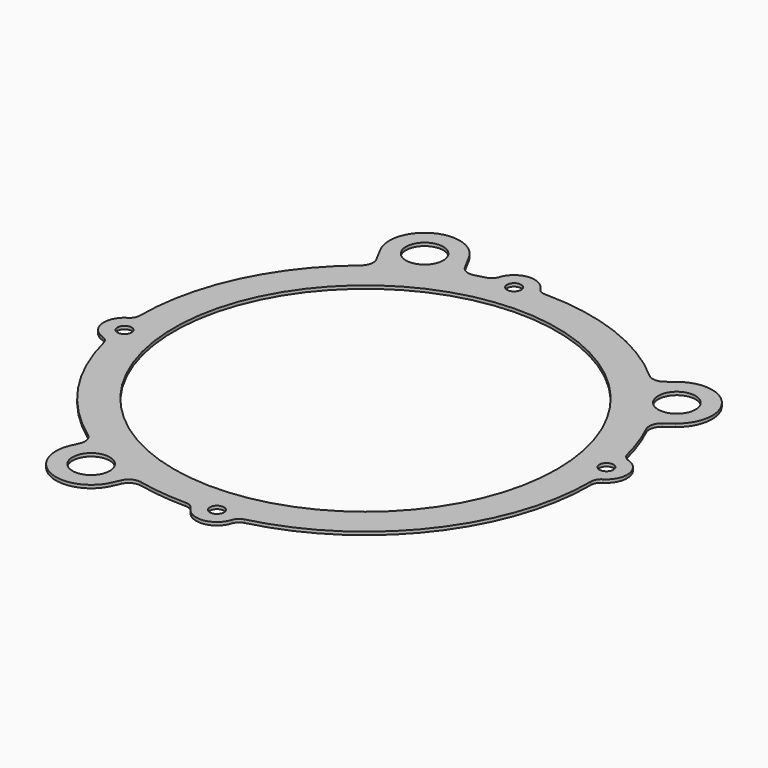
from build123d import *

# Parameters (mm, degrees)
F0_R     = 9
F0_R_2   = 3.4
F0_R_3   = 92.5
F1_DEPTH = 1.5
F2_R     = 6
F3_R     = 5


# Not quite as in the source:
# - a feature names something its author has since deleted; it is built from what else it names


with BuildPart() as f1:
    # F0 (on Top) → F1 (new body)
    with BuildSketch(Plane.XY):
        with BuildLine():
            ThreePointArc((-41.5612142371, 114.3762015069), (-64.5523398831, 121.4052940181), (-71.5814323943, 98.4141683721))
            Line((-71.5814323943, 98.4141683721), (-65.4484708904, 86.8797453608))
            ThreePointArc((-65.4484708904, 86.8797453608), (-98.0871820311, 47.0159251428), (-108.7201014418, -3.3958854983))
            ThreePointArc((-108.7201014418, -3.3958854983), (-115.9027148008, -14.2310639443), (-106.3121888463, -23.0067598447))
            ThreePointArc((-106.3121888463, -23.0067598447), (-89.5246549559, -61.7812969341), (-59.2286170286, -91.2335652089))
            Line((-59.2286170286, -91.2335652089), (-62.9150916983, -99.5135228831))
            ThreePointArc((-62.9150916983, -99.5135228831), (-54.2993418506, -121.9583185953), (-31.8545461384, -113.3425687477))
            Line((-31.8545461384, -113.3425687477), (-28.1680714687, -105.0626110734))
            ThreePointArc((-28.1680714687, -105.0626110734), (-12.5203677417, -108.0501406174), (3.3958854983, -108.7201014418))
            ThreePointArc((3.3958854983, -108.7201014418), (14.2310639443, -115.9027148008), (23.0067598447, -106.3121888463))
            ThreePointArc((23.0067598447, -106.3121888463), (85.7143913832, -66.9674219725), (108.7201014418, 3.3958854983))
            ThreePointArc((108.7201014418, 3.3958854983), (115.9027148008, 14.2310639443), (106.3121888463, 23.0067598447))
            ThreePointArc((106.3121888463, 23.0067598447), (102.1418848281, 37.3982333755), (96.0334257824, 51.0800707549))
            Line((96.0334257824, 51.0800707549), (104.0705278241, 57.1364615496))
            ThreePointArc((104.0705278241, 57.1364615496), (107.4164761014, 80.944120614), (83.608817037, 84.2900688912))
            Line((83.608817037, 84.2900688912), (75.5717149953, 78.2336780965))
            ThreePointArc((75.5717149953, 78.2336780965), (39.1751591317, 101.4736389554), (-3.3958854983, 108.7201014418))
            ThreePointArc((-3.3958854983, 108.7201014418), (-14.2310639443, 115.9027148008), (-23.0067598447, 106.3121888463))
            ThreePointArc((-23.0067598447, 106.3121888463), (-29.2689871835, 104.7612470577), (-35.4282527332, 102.8417784955))
            Line((-35.4282527332, 102.8417784955), (-41.5612142371, 114.3762015069))
        make_face()
        with Locations((-47.3848189183, -106.4280458154)):
            Circle(F0_R, mode=Mode.SUBTRACT)
        with Locations((-105.9772532844, -13.0123705102)):
            Circle(F0_R_2, mode=Mode.SUBTRACT)
        with Locations((13.0123705102, -105.9772532844)):
            Circle(F0_R_2, mode=Mode.SUBTRACT)
        Circle(F0_R_3, mode=Mode.SUBTRACT)
        with Locations((-56.5713233157, 106.3951849395)):
            Circle(F0_R, mode=Mode.SUBTRACT)
        with Locations((-13.0123705102, 105.9772532844)):
            Circle(F0_R_2, mode=Mode.SUBTRACT)
        with Locations((105.9772532844, 13.0123705102)):
            Circle(F0_R_2, mode=Mode.SUBTRACT)
        with Locations((93.8396724306, 70.7132652204)):
            Circle(F0_R, mode=Mode.SUBTRACT)
    extrude(amount=F1_DEPTH)

    # F2
    f2_edges = [f1.edges().sort_by_distance(p)[0] for p in [
        (-65.448471, 86.879745, 0.75),
        (-59.228617, -91.233565, 0.75),
        (-28.168071, -105.062611, 0.75),
        (96.033426, 51.080071, 0.75),
        (75.571715, 78.233678, 0.75),
        (-35.428253, 102.841778, 0.75),
    ]]
    fillet(f2_edges, radius=F2_R)

    # F3
    f3_edges = [f1.edges().sort_by_distance(p)[0] for p in [
        (-108.720101, -3.395885, 0.75),
        (-106.312189, -23.00676, 0.75),
        (-23.00676, 106.312189, 0.75),
        (-3.395885, 108.720101, 0.75),
        (3.395885, -108.720101, 0.75),
        (23.00676, -106.312189, 0.75),
        (108.720101, 3.395885, 0.75),
        (106.312189, 23.00676, 0.75),
    ]]
    fillet(f3_edges, radius=F3_R)


solid = f1.part
